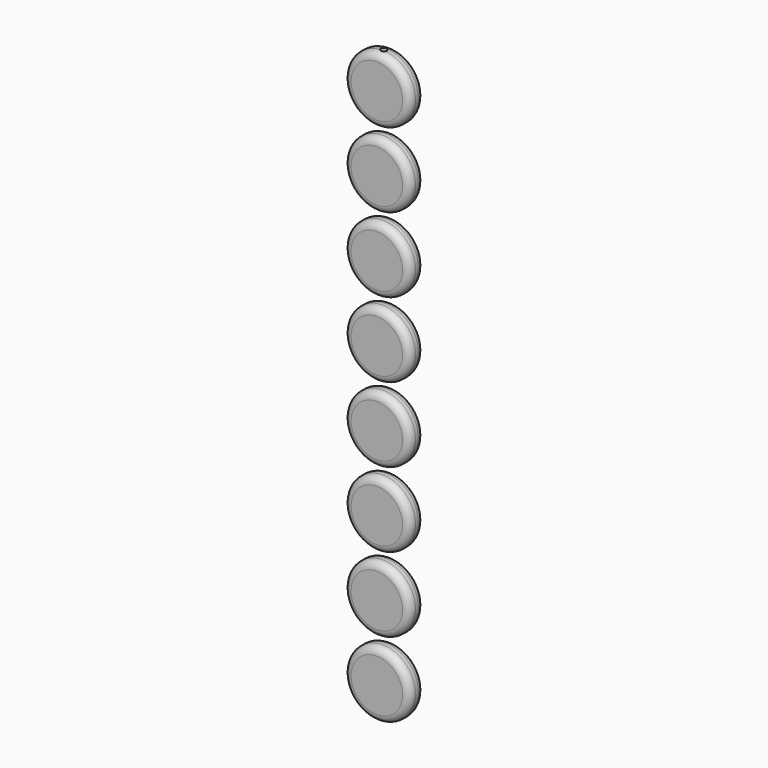
from build123d import *

# Parameters (mm, degrees)
F0_R          = 11
F1_DEPTH      = 6
F2_R          = 2.4
F2_2_R        = 2.4
F2_3_R        = 2.4
F2_4_R        = 2.4
F2_5_R        = 2.4
F2_6_R        = 2.4
F2_7_R        = 2.4
F2_8_R        = 2.4
F4_DEPTH      = 186.001
F4_DEPTH_BACK = 11.0010001


with BuildPart() as f1:
    # F0 (on Front) → F1 (new body)
    with BuildSketch(Plane.XZ):
        Circle(F0_R)
    extrude(amount=F1_DEPTH)

    # F2
    f2_edges = [f1.edges().sort_by_distance(p)[0] for p in [
        (-11, 0, 0),
        (-11, -6, 0),
    ]]
    fillet(f2_edges, radius=F2_R)

    # F3 (on Top) → F4 (cut, two sides)
    with BuildSketch(Plane.XY) as f4_sk:
        with BuildLine():
            ThreePointArc((0, -2.0515482649), (-0.7071067812, -3.7586550461), (1, -3.0515482649))
            ThreePointArc((1, -3.0515482649), (0.7071067812, -2.3444414837), (0, -2.0515482649))
        make_face()
    extrude(amount=-F4_DEPTH, mode=Mode.SUBTRACT)
    extrude(f4_sk.sketch, amount=F4_DEPTH_BACK, mode=Mode.SUBTRACT)


with BuildPart() as f1b:
    # F0 (on Front) → F1, piece 2 (new body)
    with BuildSketch(Plane.XZ):
        with Locations((0, -25)):
            Circle(F0_R)
    extrude(amount=F1_DEPTH)

    # F2#2
    f2_2_edges = [f1b.edges().sort_by_distance(p)[0] for p in [
        (-11, -6, -25),
        (-11, 0, -25),
    ]]
    fillet(f2_2_edges, radius=F2_2_R)


with BuildPart() as f1c:
    # F0 (on Front) → F1, piece 3 (new body)
    with BuildSketch(Plane.XZ):
        with Locations((0, -50)):
            Circle(F0_R)
    extrude(amount=F1_DEPTH)

    # F2#3
    f2_3_edges = [f1c.edges().sort_by_distance(p)[0] for p in [
        (-11, -6, -50),
        (-11, 0, -50),
    ]]
    fillet(f2_3_edges, radius=F2_3_R)


with BuildPart() as f1d:
    # F0 (on Front) → F1, piece 4 (new body)
    with BuildSketch(Plane.XZ):
        with Locations((0, -75)):
            Circle(F0_R)
    extrude(amount=F1_DEPTH)

    # F2#4
    f2_4_edges = [f1d.edges().sort_by_distance(p)[0] for p in [
        (-11, -6, -75),
        (-11, 0, -75),
    ]]
    fillet(f2_4_edges, radius=F2_4_R)


with BuildPart() as f1e:
    # F0 (on Front) → F1, piece 5 (new body)
    with BuildSketch(Plane.XZ):
        with Locations((0, -100)):
            Circle(F0_R)
    extrude(amount=F1_DEPTH)

    # F2#5
    f2_5_edges = [f1e.edges().sort_by_distance(p)[0] for p in [
        (-11, -6, -100),
        (-11, 0, -100),
    ]]
    fillet(f2_5_edges, radius=F2_5_R)


with BuildPart() as f1f:
    # F0 (on Front) → F1, piece 6 (new body)
    with BuildSketch(Plane.XZ):
        with Locations((0, -125)):
            Circle(F0_R)
    extrude(amount=F1_DEPTH)

    # F2#6
    f2_6_edges = [f1f.edges().sort_by_distance(p)[0] for p in [
        (-11, -6, -125),
        (-11, 0, -125),
    ]]
    fillet(f2_6_edges, radius=F2_6_R)


with BuildPart() as f1g:
    # F0 (on Front) → F1, piece 7 (new body)
    with BuildSketch(Plane.XZ):
        with Locations((0, -150)):
            Circle(F0_R)
    extrude(amount=F1_DEPTH)

    # F2#7
    f2_7_edges = [f1g.edges().sort_by_distance(p)[0] for p in [
        (-11, -6, -150),
        (-11, 0, -150),
    ]]
    fillet(f2_7_edges, radius=F2_7_R)


with BuildPart() as f1h:
    # F0 (on Front) → F1, piece 8 (new body)
    with BuildSketch(Plane.XZ):
        with Locations((0, -175)):
            Circle(F0_R)
    extrude(amount=F1_DEPTH)

    # F2#8
    f2_8_edges = [f1h.edges().sort_by_distance(p)[0] for p in [
        (-11, -6, -175),
        (-11, 0, -175),
    ]]
    fillet(f2_8_edges, radius=F2_8_R)


solid = Compound([f1.part, f1b.part, f1c.part, f1d.part, f1e.part, f1f.part, f1g.part, f1h.part])
